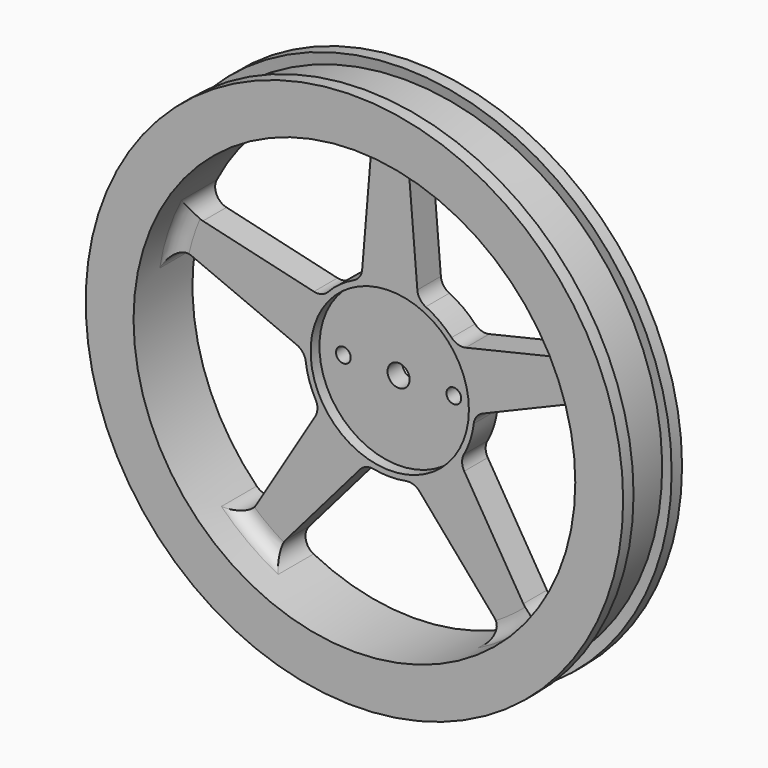
from build123d import *

# Parameters (mm, degrees)
F0_R          = 36.5
F0_R_2        = 30
F1_DEPTH      = 10
F2_R          = 11.5
F2_R_2        = 1
F2_R_3        = 1.5
F3_DEPTH      = 4
F5_DEPTH      = 4
F6_T1_DEPTH   = 4
F6_T6_ANGLE   = 27.7282501568
F6_T12_ANGLE  = 27.7282501568
F6_T18_ANGLE  = 27.7282501568
F6_T24_ANGLE  = 27.7282501568
F6_T30_ANGLE  = 27.7282501568
F6_T37_ANGLE  = 27.7282501568
F6_T41_DEPTH  = 10.3294220662
F6_T49_DEPTH  = 10.3294220662
F6_T54_ANGLE  = 27.7282501568
F6_T61_ANGLE  = 27.7282501568
F6_T65_DEPTH  = 10.3294220662
F6_T73_DEPTH  = 10.3294220662
F6_T78_ANGLE  = 27.7282501568
F6_T85_ANGLE  = 27.7282501568
F6_T89_DEPTH  = 10.3294220662
F6_T97_DEPTH  = 10.3294220662
F6_T102_ANGLE = 27.7282501568
F6_T109_ANGLE = 27.7282501568
F6_T113_DEPTH = 10.3294220662
F6_T121_DEPTH = 10.3294220662
F6_T126_ANGLE = 27.7282501568
F6_T133_ANGLE = 27.7282501568
F6_T137_DEPTH = 10.3294220662
F6_T145_DEPTH = 10.3294220662
F6_T150_ANGLE = 27.7282501568
F7_R          = 10.75
F8_DEPTH      = 1.5


# Not quite as in the source:
# - a fillet or chamfer that OpenCascade refuses, or shapes differently, is made with other operations: its cross-section is extruded or revolved along the edge and cut away or added
# - a feature names something its author has since deleted; it is built from what else it names


with BuildPart() as f1:
    # F0 (on Front) → F1 (new body)
    with BuildSketch(Plane.XZ):
        Circle(F0_R)
        Circle(F0_R_2, mode=Mode.SUBTRACT)
    extrude(amount=F1_DEPTH)



with BuildPart() as f3:
    # F2 (on Front) → F3 (new body)
    with BuildSketch(Plane.XZ):
        Circle(F2_R)
        with Locations((-7.5, 0)):
            Circle(F2_R_2, mode=Mode.SUBTRACT)
        Circle(F2_R_3, mode=Mode.SUBTRACT)
        with Locations((7.5, 0)):
            Circle(F2_R_2, mode=Mode.SUBTRACT)
    extrude(amount=F3_DEPTH)


with BuildPart() as f1_1:
    add(f1.part)

    add(f3.part)  # F5 merges F3
    # F4 (on Front) → F5 (join)
    with BuildSketch(Plane.XZ):
        Polygon((-2, 33), (-4, 9), (4, 9), (2, 33), align=None)
        Polygon((-30.766831049, 12.099673847), (-32.0028990265, 8.2954477818), (-9.7955766242, -1.0230731158), (-7.3234406692, 6.5853790146), align=None)
        Polygon((-21.0149473144, -25.5219903098), (-17.7788793369, -27.873131319), (-2.0539992931, -9.6322939585), (-8.5261352481, -4.9300119402), align=None)
        Polygon((17.7788793369, -27.873131319), (21.0149473144, -25.5219903098), (8.5261352481, -4.9300119402), (2.0539992931, -9.6322939585), align=None)
        Polygon((32.0028990265, 8.2954477818), (30.766831049, 12.099673847), (7.3234406692, 6.5853790146), (9.7955766242, -1.0230731158), align=None)
    extrude(amount=F5_DEPTH)

    # F6: fillet of radius 2 on 25 edges, made by hand

    # F6_s2 → F6_t1 (join)
    with BuildSketch(Plane.XZ):
        with BuildLine():
            ThreePointArc((4.7713926974, 29.6181331574), (3.0942624237, 29.1109072971), (2.4602083344, 27.4774999872))
            Line((2.4602083344, 27.4774999872), (2.2570856463, 29.9149722444))
            ThreePointArc((2.2570856463, 29.9149722444), (3.5173719334, 29.7930880354), (4.7713926974, 29.6181331574))
        make_face()
        with BuildLine():
            ThreePointArc((-4.7713926974, 29.6181331574), (-3.0942624237, 29.1109072971), (-2.4602083344, 27.4774999872))
            Line((-2.4602083344, 27.4774999872), (-2.2570856463, 29.9149722444))
            ThreePointArc((-2.2570856463, 29.9149722444), (-3.5173719334, 29.7930880354), (-4.7713926974, 29.6181331574))
        make_face()
        with BuildLine():
            ThreePointArc((-13.5489640913, -26.7661273264), (-14.6076511042, -25.3699805444), (-14.1605189101, -23.6758386291))
            Line((-14.1605189101, -23.6758386291), (-15.7575588624, -25.5284025881))
            ThreePointArc((-15.7575588624, -25.5284025881), (-14.6663240978, -26.1705738848), (-13.5489640913, -26.7661273264))
        make_face()
        with BuildLine():
            ThreePointArc((-26.6940771095, 13.6903706039), (-26.7299384062, 11.9385835177), (-25.3724092293, 10.8308116268))
            Line((-25.3724092293, 10.8308116268), (-27.7533514654, 11.3908508215))
            ThreePointArc((-27.7533514654, 11.3908508215), (-27.2479828136, 12.5517900153), (-26.6940771095, 13.6903706039))
        make_face()
        with BuildLine():
            ThreePointArc((-29.6429599701, 4.6146423706), (-28.6422977541, 6.0529466353), (-26.8929015993, 6.1512172911))
            Line((-26.8929015993, 6.1512172911), (-29.1483071103, 7.097618798))
            ThreePointArc((-29.1483071103, 7.097618798), (-29.4218382195, 5.8613510203), (-29.6429599701, 4.6146423706))
        make_face()
        with BuildLine():
            ThreePointArc((-21.2692396494, -21.1570188055), (-19.6142728759, -21.7324569056), (-18.1412196146, -20.783690276))
            Line((-18.1412196146, -20.783690276), (-19.4096001536, -22.8750392759))
            ThreePointArc((-19.4096001536, -22.8750392759), (-20.3575514371, -22.0356551862), (-21.2692396494, -21.1570188055))
        make_face()
        with BuildLine():
            ThreePointArc((-4.054653915, -11.9530503313), (-3.1974418623, -11.3701338379), (-2.1635629978, -11.2946445342))
            ThreePointArc((-2.1635629978, -11.2946445342), (-2.7140069187, -11.1751584528), (-3.2579399845, -11.028863362))
            Line((-3.2579399845, -11.028863362), (-4.054653915, -11.9530503313))
        make_face()
        with BuildLine():
            ThreePointArc((-10.1150694411, -7.5499007142), (-9.8255760037, -6.5545125029), (-10.0732675488, -5.547907794))
            ThreePointArc((-10.0732675488, -5.547907794), (-9.7895330065, -6.034487842), (-9.4823135459, -6.5065912594))
            Line((-9.4823135459, -6.5065912594), (-10.1150694411, -7.5499007142))
        make_face()
        with BuildLine():
            ThreePointArc((-12.6209833732, 0.1625093402), (-11.8017037517, -0.4726166656), (-11.4104230182, -1.432566419))
            ThreePointArc((-11.4104230182, -1.432566419), (-11.4668815279, -0.8721399115), (-11.4958311896, -0.3096211556))
            Line((-11.4958311896, -0.3096211556), (-12.6209833732, 0.1625093402))
        make_face()
        with BuildLine():
            ThreePointArc((-10.3061106282, 7.2869550782), (-9.2699817917, 7.3192223314), (-8.3891847207, 7.8658489511))
            ThreePointArc((-8.3891847207, 7.8658489511), (-8.7642710506, 7.4456398617), (-9.1183320478, 7.0075688128))
            Line((-9.1183320478, 7.0075688128), (-10.3061106282, 7.2869550782))
        make_face()
        with BuildLine():
            ThreePointArc((-3.7455427811, 12.053486627), (-4.0964121814, 11.0780406749), (-4.8884662535, 10.4092697961))
            ThreePointArc((-4.8884662535, 10.4092697961), (-4.3729156105, 10.6361463446), (-3.8468744196, 10.8375069642))
            Line((-3.8468744196, 10.8375069642), (-3.7455427811, 12.053486627))
        make_face()
        with BuildLine():
            ThreePointArc((3.7455427811, 12.053486627), (4.0964121814, 11.0780406749), (4.8884662535, 10.4092697961))
            ThreePointArc((4.8884662535, 10.4092697961), (4.3729156105, 10.6361463446), (3.8468744196, 10.8375069642))
            Line((3.8468744196, 10.8375069642), (3.7455427811, 12.053486627))
        make_face()
        with BuildLine():
            ThreePointArc((29.6429599701, 4.6146423706), (28.6422977541, 6.0529466353), (26.8929015993, 6.1512172911))
            Line((26.8929015993, 6.1512172911), (29.1483071103, 7.097618798))
            ThreePointArc((29.1483071103, 7.097618798), (29.4218382195, 5.8613510203), (29.6429599701, 4.6146423706))
        make_face()
        with BuildLine():
            ThreePointArc((26.6940771095, 13.6903706039), (26.7299384062, 11.9385835177), (25.3724092293, 10.8308116268))
            Line((25.3724092293, 10.8308116268), (27.7533514654, 11.3908508215))
            ThreePointArc((27.7533514654, 11.3908508215), (27.2479828136, 12.5517900153), (26.6940771095, 13.6903706039))
        make_face()
        with BuildLine():
            ThreePointArc((13.5489640913, -26.7661273264), (14.6076511042, -25.3699805444), (14.1605189101, -23.6758386291))
            Line((14.1605189101, -23.6758386291), (15.7575588624, -25.5284025881))
            ThreePointArc((15.7575588624, -25.5284025881), (14.6663240978, -26.1705738848), (13.5489640913, -26.7661273264))
        make_face()
        with BuildLine():
            ThreePointArc((21.2692396494, -21.1570188055), (19.6142728759, -21.7324569056), (18.1412196146, -20.783690276))
            Line((18.1412196146, -20.783690276), (19.4096001536, -22.8750392759))
            ThreePointArc((19.4096001536, -22.8750392759), (20.3575514371, -22.0356551862), (21.2692396494, -21.1570188055))
        make_face()
        with BuildLine():
            ThreePointArc((12.6209833732, 0.1625093402), (11.8017037517, -0.4726166656), (11.4104230182, -1.432566419))
            ThreePointArc((11.4104230182, -1.432566419), (11.4668815279, -0.8721399115), (11.4958311896, -0.3096211556))
            Line((11.4958311896, -0.3096211556), (12.6209833732, 0.1625093402))
        make_face()
        with BuildLine():
            ThreePointArc((10.3061106282, 7.2869550782), (9.2699817917, 7.3192223314), (8.3891847207, 7.8658489511))
            ThreePointArc((8.3891847207, 7.8658489511), (8.7642710506, 7.4456398617), (9.1183320478, 7.0075688128))
            Line((9.1183320478, 7.0075688128), (10.3061106282, 7.2869550782))
        make_face()
        with BuildLine():
            ThreePointArc((4.054653915, -11.9530503313), (3.1974418623, -11.3701338379), (2.1635629978, -11.2946445342))
            ThreePointArc((2.1635629978, -11.2946445342), (2.7140069187, -11.1751584528), (3.2579399845, -11.028863362))
            Line((3.2579399845, -11.028863362), (4.054653915, -11.9530503313))
        make_face()
        with BuildLine():
            ThreePointArc((10.1150694411, -7.5499007142), (9.8255760037, -6.5545125029), (10.0732675488, -5.547907794))
            ThreePointArc((10.0732675488, -5.547907794), (9.7895330065, -6.034487842), (9.4823135459, -6.5065912594))
            Line((9.4823135459, -6.5065912594), (10.1150694411, -7.5499007142))
        make_face()
    extrude(amount=F6_T1_DEPTH)


with BuildPart() as f6_tool4:
    # F6_s5 → F6_t6 (revolve)
    with BuildSketch(Plane(origin=(0, 0, 0), x_dir=(0, 1, 0), z_dir=(-0.5279066599, 0, 0.8493023952))):
        with BuildLine():
            ThreePointArc((-6, -30), (-4.5857864376, -29.4142135624), (-4, -28))
            Line((-4, -28), (-4, -30))
            Line((-4, -30), (-6, -30))
        make_face()
    revolve(axis=Axis((0, -4, 0), (0, 1, 0)), revolution_arc=F6_T6_ANGLE)

    split(bisect_by=Plane(origin=(1.8315713488, 0, -4.3648875067), x_dir=(0, 1, 0), z_dir=(-0.3869305197, 0, 0.9221088726)), keep=Keep.TOP)

    split(bisect_by=Plane(origin=(-1.0838441567, 0, 4.6078387988), x_dir=(0, 1, 0), z_dir=(0.2289686302, 0, -0.9734338017)), keep=Keep.TOP)


with BuildPart() as f1_2:
    add(f1_1.part)

    # F6_t3: union F6_tool4
    add(f6_tool4.part)


with BuildPart() as f6_tool10:
    # F6_s11 → F6_t12 (revolve)
    with BuildSketch(Plane(origin=(0, 0, 0), x_dir=(0, 1, 0), z_dir=(-0.9708667066, 0, -0.2396201954))):
        with BuildLine():
            ThreePointArc((-6, -30), (-4.5857864376, -29.4142135624), (-4, -28))
            Line((-4, -28), (-4, -30))
            Line((-4, -30), (-6, -30))
        make_face()
    revolve(axis=Axis((0, -4, 0), (0, 1, 0)), revolution_arc=F6_T12_ANGLE)

    split(bisect_by=Plane(origin=(4.7172413793, 0, 0.3931034483), x_dir=(0, 1, 0), z_dir=(-0.9965457582, 0, -0.0830454799)), keep=Keep.TOP)

    split(bisect_by=Plane(origin=(-4.7172413793, 0, 0.3931034483), x_dir=(0, 1, 0), z_dir=(0.9965457582, 0, -0.0830454799)), keep=Keep.TOP)


with BuildPart() as f1_3:
    add(f1_2.part)

    # F6_t9: union F6_tool10
    add(f6_tool10.part)


with BuildPart() as f6_tool16:
    # F6_s17 → F6_t18 (revolve)
    with BuildSketch(Plane(origin=(0, 0, 0), x_dir=(0, 1, 0), z_dir=(-0.0721219634, 0, -0.9973958203))):
        with BuildLine():
            ThreePointArc((-6, -30), (-4.5857864376, -29.4142135624), (-4, -28))
            Line((-4, -28), (-4, -30))
            Line((-4, -30), (-6, -30))
        make_face()
    revolve(axis=Axis((0, -4, 0), (0, 1, 0)), revolution_arc=F6_T18_ANGLE)

    split(bisect_by=Plane(origin=(1.0838441567, 0, 4.6078387988), x_dir=(0, 1, 0), z_dir=(-0.2289686302, 0, -0.9734338017)), keep=Keep.TOP)

    split(bisect_by=Plane(origin=(-1.8315713488, 0, -4.3648875067), x_dir=(0, 1, 0), z_dir=(0.3869305197, 0, 0.9221088726)), keep=Keep.TOP)


with BuildPart() as f1_4:
    add(f1_3.part)

    # F6_t15: union F6_tool16
    add(f6_tool16.part)


with BuildPart() as f6_tool22:
    # F6_s23 → F6_t24 (revolve)
    with BuildSketch(Plane(origin=(0, 0, 0), x_dir=(0, 1, 0), z_dir=(0.9262928819, 0, -0.3768043218))):
        with BuildLine():
            ThreePointArc((-6, -30), (-4.5857864376, -29.4142135624), (-4, -28))
            Line((-4, -28), (-4, -30))
            Line((-4, -30), (-6, -30))
        make_face()
    revolve(axis=Axis((0, -4, 0), (0, 1, 0)), revolution_arc=F6_T24_ANGLE)

    split(bisect_by=Plane(origin=(-4.047388852, 0, 2.4546975441), x_dir=(0, 1, 0), z_dir=(0.8550353624, 0, -0.5185696954)), keep=Keep.TOP)

    split(bisect_by=Plane(origin=(3.5852680329, 0, -3.0907522845), x_dir=(0, 1, 0), z_dir=(-0.7574095458, 0, 0.6529401044)), keep=Keep.TOP)


with BuildPart() as f1_5:
    add(f1_4.part)

    # F6_t21: union F6_tool22
    add(f6_tool22.part)


with BuildPart() as f6_tool28:
    # F6_s29 → F6_t30 (revolve)
    with BuildSketch(Plane(origin=(0, 0, 0), x_dir=(0, 1, 0), z_dir=(0.6446024479, 0, 0.7645179423))):
        with BuildLine():
            ThreePointArc((-6, -30), (-4.5857864376, -29.4142135624), (-4, -28))
            Line((-4, -28), (-4, -30))
            Line((-4, -30), (-6, -30))
        make_face()
    revolve(axis=Axis((0, -4, 0), (0, 1, 0)), revolution_arc=F6_T30_ANGLE)

    split(bisect_by=Plane(origin=(-3.5852680329, 0, -3.0907522845), x_dir=(0, 1, 0), z_dir=(0.7574095458, 0, 0.6529401044)), keep=Keep.TOP)

    split(bisect_by=Plane(origin=(4.047388852, 0, 2.4546975441), x_dir=(0, 1, 0), z_dir=(-0.8550353624, 0, -0.5185696954)), keep=Keep.TOP)


with BuildPart() as f1_6:
    add(f1_5.part)

    # F6_t27: union F6_tool28
    add(f6_tool28.part)


with BuildPart() as f6_tool35:
    # F6_s36 → F6_t37 (revolve)
    with BuildSketch(Plane(origin=(0, 0, 0), x_dir=(0, 1, 0), z_dir=(-0.5279066599, 0, 0.8493023952))):
        with BuildLine():
            ThreePointArc((-6, -30), (-4.5857864376, -29.4142135624), (-4, -28))
            Line((-4, -28), (-4, -30))
            Line((-4, -30), (-6, -30))
        make_face()
    revolve(axis=Axis((0, -4, 0), (0, 1, 0)), revolution_arc=F6_T37_ANGLE)

    split(bisect_by=Plane(origin=(-1.0838441567, 0, 4.6078387988), x_dir=(0, 1, 0), z_dir=(-0.2289686302, 0, 0.9734338017)), keep=Keep.TOP)


with BuildPart() as f6_tool39:
    # F6_s40 → F6_t41 (new body)
    with BuildSketch(Plane.XZ.offset(10.3294220662)):
        with BuildLine():
            ThreePointArc((26.6940771095, 13.6903706039), (26.7299384062, 11.9385835177), (25.3724092293, 10.8308116268))
            Line((25.3724092293, 10.8308116268), (27.7533514654, 11.3908508215))
            ThreePointArc((27.7533514654, 11.3908508215), (27.2479828136, 12.5517900153), (26.6940771095, 13.6903706039))
        make_face()
    extrude(amount=-F6_T41_DEPTH)

    split(bisect_by=Plane.XZ.offset(10), keep=Keep.BOTTOM)

    split(bisect_by=Plane.XZ.offset(4), keep=Keep.TOP)


with BuildPart() as f6_tool35_1:
    add(f6_tool35.part)

    # F6_t44: intersect F6_tool39
    add(f6_tool39.part, mode=Mode.INTERSECT)


with BuildPart() as f1_7:
    add(f1_6.part)

    # F6_t33: union F6_tool35
    add(f6_tool35_1.part)


with BuildPart() as f6_tool47:
    # F6_s48 → F6_t49 (new body)
    with BuildSketch(Plane.XZ.offset(10.3294220662)):
        with BuildLine():
            ThreePointArc((29.6429599701, 4.6146423706), (28.6422977541, 6.0529466353), (26.8929015993, 6.1512172911))
            Line((26.8929015993, 6.1512172911), (29.1483071103, 7.097618798))
            ThreePointArc((29.1483071103, 7.097618798), (29.4218382195, 5.8613510203), (29.6429599701, 4.6146423706))
        make_face()
    extrude(amount=-F6_T49_DEPTH)

    split(bisect_by=Plane.XZ.offset(10), keep=Keep.BOTTOM)

    split(bisect_by=Plane.XZ.offset(4), keep=Keep.TOP)


with BuildPart() as f6_tool52:
    # F6_s53 → F6_t54 (revolve)
    with BuildSketch(Plane(origin=(0, 0, 0), x_dir=(0, 1, 0), z_dir=(-0.5279066599, 0, 0.8493023952))):
        with BuildLine():
            ThreePointArc((-6, -30), (-4.5857864376, -29.4142135624), (-4, -28))
            Line((-4, -28), (-4, -30))
            Line((-4, -30), (-6, -30))
        make_face()
    revolve(axis=Axis((0, -4, 0), (0, 1, 0)), revolution_arc=F6_T54_ANGLE)

    split(bisect_by=Plane(origin=(1.8315713488, 0, -4.3648875067), x_dir=(0, 1, 0), z_dir=(0.3869305197, 0, -0.9221088726)), keep=Keep.TOP)


with BuildPart() as f6_tool47_1:
    add(f6_tool47.part)

    # F6_t56: intersect F6_tool52
    add(f6_tool52.part, mode=Mode.INTERSECT)


with BuildPart() as f1_8:
    add(f1_7.part)

    # F6_t45: union F6_tool47
    add(f6_tool47_1.part)


with BuildPart() as f6_tool59:
    # F6_s60 → F6_t61 (revolve)
    with BuildSketch(Plane(origin=(0, 0, 0), x_dir=(0, 1, 0), z_dir=(-0.9708667066, 0, -0.2396201954))):
        with BuildLine():
            ThreePointArc((-6, -30), (-4.5857864376, -29.4142135624), (-4, -28))
            Line((-4, -28), (-4, -30))
            Line((-4, -30), (-6, -30))
        make_face()
    revolve(axis=Axis((0, -4, 0), (0, 1, 0)), revolution_arc=F6_T61_ANGLE)

    split(bisect_by=Plane(origin=(-4.7172413793, 0, 0.3931034483), x_dir=(0, 1, 0), z_dir=(-0.9965457582, 0, 0.0830454799)), keep=Keep.TOP)


with BuildPart() as f6_tool63:
    # F6_s64 → F6_t65 (new body)
    with BuildSketch(Plane.XZ.offset(10.3294220662)):
        with BuildLine():
            ThreePointArc((-4.7713926974, 29.6181331574), (-3.0942624237, 29.1109072971), (-2.4602083344, 27.4774999872))
            Line((-2.4602083344, 27.4774999872), (-2.2570856463, 29.9149722444))
            ThreePointArc((-2.2570856463, 29.9149722444), (-3.5173719334, 29.7930880354), (-4.7713926974, 29.6181331574))
        make_face()
    extrude(amount=-F6_T65_DEPTH)

    split(bisect_by=Plane.XZ.offset(10), keep=Keep.BOTTOM)

    split(bisect_by=Plane.XZ.offset(4), keep=Keep.TOP)


with BuildPart() as f6_tool59_1:
    add(f6_tool59.part)

    # F6_t68: intersect F6_tool63
    add(f6_tool63.part, mode=Mode.INTERSECT)


with BuildPart() as f1_9:
    add(f1_8.part)

    # F6_t57: union F6_tool59
    add(f6_tool59_1.part)


with BuildPart() as f6_tool71:
    # F6_s72 → F6_t73 (new body)
    with BuildSketch(Plane.XZ.offset(10.3294220662)):
        with BuildLine():
            ThreePointArc((4.7713926974, 29.6181331574), (3.0942624237, 29.1109072971), (2.4602083344, 27.4774999872))
            Line((2.4602083344, 27.4774999872), (2.2570856463, 29.9149722444))
            ThreePointArc((2.2570856463, 29.9149722444), (3.5173719334, 29.7930880354), (4.7713926974, 29.6181331574))
        make_face()
    extrude(amount=-F6_T73_DEPTH)

    split(bisect_by=Plane.XZ.offset(10), keep=Keep.BOTTOM)

    split(bisect_by=Plane.XZ.offset(4), keep=Keep.TOP)


with BuildPart() as f6_tool76:
    # F6_s77 → F6_t78 (revolve)
    with BuildSketch(Plane(origin=(0, 0, 0), x_dir=(0, 1, 0), z_dir=(-0.9708667066, 0, -0.2396201954))):
        with BuildLine():
            ThreePointArc((-6, -30), (-4.5857864376, -29.4142135624), (-4, -28))
            Line((-4, -28), (-4, -30))
            Line((-4, -30), (-6, -30))
        make_face()
    revolve(axis=Axis((0, -4, 0), (0, 1, 0)), revolution_arc=F6_T78_ANGLE)

    split(bisect_by=Plane(origin=(4.7172413793, 0, 0.3931034483), x_dir=(0, 1, 0), z_dir=(0.9965457582, 0, 0.0830454799)), keep=Keep.TOP)


with BuildPart() as f6_tool71_1:
    add(f6_tool71.part)

    # F6_t80: intersect F6_tool76
    add(f6_tool76.part, mode=Mode.INTERSECT)


with BuildPart() as f1_10:
    add(f1_9.part)

    # F6_t69: union F6_tool71
    add(f6_tool71_1.part)


with BuildPart() as f6_tool83:
    # F6_s84 → F6_t85 (revolve)
    with BuildSketch(Plane(origin=(0, 0, 0), x_dir=(0, 1, 0), z_dir=(-0.0721219634, 0, -0.9973958203))):
        with BuildLine():
            ThreePointArc((-6, -30), (-4.5857864376, -29.4142135624), (-4, -28))
            Line((-4, -28), (-4, -30))
            Line((-4, -30), (-6, -30))
        make_face()
    revolve(axis=Axis((0, -4, 0), (0, 1, 0)), revolution_arc=F6_T85_ANGLE)

    split(bisect_by=Plane(origin=(-1.8315713488, 0, -4.3648875067), x_dir=(0, 1, 0), z_dir=(-0.3869305197, 0, -0.9221088726)), keep=Keep.TOP)


with BuildPart() as f6_tool87:
    # F6_s88 → F6_t89 (new body)
    with BuildSketch(Plane.XZ.offset(10.3294220662)):
        with BuildLine():
            ThreePointArc((-29.6429599701, 4.6146423706), (-28.6422977541, 6.0529466353), (-26.8929015993, 6.1512172911))
            Line((-26.8929015993, 6.1512172911), (-29.1483071103, 7.097618798))
            ThreePointArc((-29.1483071103, 7.097618798), (-29.4218382195, 5.8613510203), (-29.6429599701, 4.6146423706))
        make_face()
    extrude(amount=-F6_T89_DEPTH)

    split(bisect_by=Plane.XZ.offset(10), keep=Keep.BOTTOM)

    split(bisect_by=Plane.XZ.offset(4), keep=Keep.TOP)


with BuildPart() as f6_tool83_1:
    add(f6_tool83.part)

    # F6_t92: intersect F6_tool87
    add(f6_tool87.part, mode=Mode.INTERSECT)


with BuildPart() as f1_11:
    add(f1_10.part)

    # F6_t81: union F6_tool83
    add(f6_tool83_1.part)


with BuildPart() as f6_tool95:
    # F6_s96 → F6_t97 (new body)
    with BuildSketch(Plane.XZ.offset(10.3294220662)):
        with BuildLine():
            ThreePointArc((-26.6940771095, 13.6903706039), (-26.7299384062, 11.9385835177), (-25.3724092293, 10.8308116268))
            Line((-25.3724092293, 10.8308116268), (-27.7533514654, 11.3908508215))
            ThreePointArc((-27.7533514654, 11.3908508215), (-27.2479828136, 12.5517900153), (-26.6940771095, 13.6903706039))
        make_face()
    extrude(amount=-F6_T97_DEPTH)

    split(bisect_by=Plane.XZ.offset(10), keep=Keep.BOTTOM)

    split(bisect_by=Plane.XZ.offset(4), keep=Keep.TOP)


with BuildPart() as f6_tool100:
    # F6_s101 → F6_t102 (revolve)
    with BuildSketch(Plane(origin=(0, 0, 0), x_dir=(0, 1, 0), z_dir=(-0.0721219634, 0, -0.9973958203))):
        with BuildLine():
            ThreePointArc((-6, -30), (-4.5857864376, -29.4142135624), (-4, -28))
            Line((-4, -28), (-4, -30))
            Line((-4, -30), (-6, -30))
        make_face()
    revolve(axis=Axis((0, -4, 0), (0, 1, 0)), revolution_arc=F6_T102_ANGLE)

    split(bisect_by=Plane(origin=(1.0838441567, 0, 4.6078387988), x_dir=(0, 1, 0), z_dir=(0.2289686302, 0, 0.9734338017)), keep=Keep.TOP)


with BuildPart() as f6_tool95_1:
    add(f6_tool95.part)

    # F6_t104: intersect F6_tool100
    add(f6_tool100.part, mode=Mode.INTERSECT)


with BuildPart() as f1_12:
    add(f1_11.part)

    # F6_t93: union F6_tool95
    add(f6_tool95_1.part)


with BuildPart() as f6_tool107:
    # F6_s108 → F6_t109 (revolve)
    with BuildSketch(Plane(origin=(0, 0, 0), x_dir=(0, 1, 0), z_dir=(0.9262928819, 0, -0.3768043218))):
        with BuildLine():
            ThreePointArc((-6, -30), (-4.5857864376, -29.4142135624), (-4, -28))
            Line((-4, -28), (-4, -30))
            Line((-4, -30), (-6, -30))
        make_face()
    revolve(axis=Axis((0, -4, 0), (0, 1, 0)), revolution_arc=F6_T109_ANGLE)

    split(bisect_by=Plane(origin=(3.5852680329, 0, -3.0907522845), x_dir=(0, 1, 0), z_dir=(0.7574095458, 0, -0.6529401044)), keep=Keep.TOP)


with BuildPart() as f6_tool111:
    # F6_s112 → F6_t113 (new body)
    with BuildSketch(Plane.XZ.offset(10.3294220662)):
        with BuildLine():
            ThreePointArc((-13.5489640913, -26.7661273264), (-14.6076511042, -25.3699805444), (-14.1605189101, -23.6758386291))
            Line((-14.1605189101, -23.6758386291), (-15.7575588624, -25.5284025881))
            ThreePointArc((-15.7575588624, -25.5284025881), (-14.6663240978, -26.1705738848), (-13.5489640913, -26.7661273264))
        make_face()
    extrude(amount=-F6_T113_DEPTH)

    split(bisect_by=Plane.XZ.offset(10), keep=Keep.BOTTOM)

    split(bisect_by=Plane.XZ.offset(4), keep=Keep.TOP)


with BuildPart() as f6_tool107_1:
    add(f6_tool107.part)

    # F6_t116: intersect F6_tool111
    add(f6_tool111.part, mode=Mode.INTERSECT)


with BuildPart() as f1_13:
    add(f1_12.part)

    # F6_t105: union F6_tool107
    add(f6_tool107_1.part)


with BuildPart() as f6_tool119:
    # F6_s120 → F6_t121 (new body)
    with BuildSketch(Plane.XZ.offset(10.3294220662)):
        with BuildLine():
            ThreePointArc((-21.2692396494, -21.1570188055), (-19.6142728759, -21.7324569056), (-18.1412196146, -20.783690276))
            Line((-18.1412196146, -20.783690276), (-19.4096001536, -22.8750392759))
            ThreePointArc((-19.4096001536, -22.8750392759), (-20.3575514371, -22.0356551862), (-21.2692396494, -21.1570188055))
        make_face()
    extrude(amount=-F6_T121_DEPTH)

    split(bisect_by=Plane.XZ.offset(10), keep=Keep.BOTTOM)

    split(bisect_by=Plane.XZ.offset(4), keep=Keep.TOP)


with BuildPart() as f6_tool124:
    # F6_s125 → F6_t126 (revolve)
    with BuildSketch(Plane(origin=(0, 0, 0), x_dir=(0, 1, 0), z_dir=(0.9262928819, 0, -0.3768043218))):
        with BuildLine():
            ThreePointArc((-6, -30), (-4.5857864376, -29.4142135624), (-4, -28))
            Line((-4, -28), (-4, -30))
            Line((-4, -30), (-6, -30))
        make_face()
    revolve(axis=Axis((0, -4, 0), (0, 1, 0)), revolution_arc=F6_T126_ANGLE)

    split(bisect_by=Plane(origin=(-4.047388852, 0, 2.4546975441), x_dir=(0, 1, 0), z_dir=(-0.8550353624, 0, 0.5185696954)), keep=Keep.TOP)


with BuildPart() as f6_tool119_1:
    add(f6_tool119.part)

    # F6_t128: intersect F6_tool124
    add(f6_tool124.part, mode=Mode.INTERSECT)


with BuildPart() as f1_14:
    add(f1_13.part)

    # F6_t117: union F6_tool119
    add(f6_tool119_1.part)


with BuildPart() as f6_tool131:
    # F6_s132 → F6_t133 (revolve)
    with BuildSketch(Plane(origin=(0, 0, 0), x_dir=(0, 1, 0), z_dir=(0.6446024479, 0, 0.7645179423))):
        with BuildLine():
            ThreePointArc((-6, -30), (-4.5857864376, -29.4142135624), (-4, -28))
            Line((-4, -28), (-4, -30))
            Line((-4, -30), (-6, -30))
        make_face()
    revolve(axis=Axis((0, -4, 0), (0, 1, 0)), revolution_arc=F6_T133_ANGLE)

    split(bisect_by=Plane(origin=(4.047388852, 0, 2.4546975441), x_dir=(0, 1, 0), z_dir=(0.8550353624, 0, 0.5185696954)), keep=Keep.TOP)


with BuildPart() as f6_tool135:
    # F6_s136 → F6_t137 (new body)
    with BuildSketch(Plane.XZ.offset(10.3294220662)):
        with BuildLine():
            ThreePointArc((21.2692396494, -21.1570188055), (19.6142728759, -21.7324569056), (18.1412196146, -20.783690276))
            Line((18.1412196146, -20.783690276), (19.4096001536, -22.8750392759))
            ThreePointArc((19.4096001536, -22.8750392759), (20.3575514371, -22.0356551862), (21.2692396494, -21.1570188055))
        make_face()
    extrude(amount=-F6_T137_DEPTH)

    split(bisect_by=Plane.XZ.offset(10), keep=Keep.BOTTOM)

    split(bisect_by=Plane.XZ.offset(4), keep=Keep.TOP)


with BuildPart() as f6_tool131_1:
    add(f6_tool131.part)

    # F6_t140: intersect F6_tool135
    add(f6_tool135.part, mode=Mode.INTERSECT)


with BuildPart() as f1_15:
    add(f1_14.part)

    # F6_t129: union F6_tool131
    add(f6_tool131_1.part)


with BuildPart() as f6_tool143:
    # F6_s144 → F6_t145 (new body)
    with BuildSketch(Plane.XZ.offset(10.3294220662)):
        with BuildLine():
            ThreePointArc((13.5489640913, -26.7661273264), (14.6076511042, -25.3699805444), (14.1605189101, -23.6758386291))
            Line((14.1605189101, -23.6758386291), (15.7575588624, -25.5284025881))
            ThreePointArc((15.7575588624, -25.5284025881), (14.6663240978, -26.1705738848), (13.5489640913, -26.7661273264))
        make_face()
    extrude(amount=-F6_T145_DEPTH)

    split(bisect_by=Plane.XZ.offset(10), keep=Keep.BOTTOM)

    split(bisect_by=Plane.XZ.offset(4), keep=Keep.TOP)


with BuildPart() as f6_tool148:
    # F6_s149 → F6_t150 (revolve)
    with BuildSketch(Plane(origin=(0, 0, 0), x_dir=(0, 1, 0), z_dir=(0.6446024479, 0, 0.7645179423))):
        with BuildLine():
            ThreePointArc((-6, -30), (-4.5857864376, -29.4142135624), (-4, -28))
            Line((-4, -28), (-4, -30))
            Line((-4, -30), (-6, -30))
        make_face()
    revolve(axis=Axis((0, -4, 0), (0, 1, 0)), revolution_arc=F6_T150_ANGLE)

    split(bisect_by=Plane(origin=(-3.5852680329, 0, -3.0907522845), x_dir=(0, 1, 0), z_dir=(-0.7574095458, 0, -0.6529401044)), keep=Keep.TOP)


with BuildPart() as f6_tool143_1:
    add(f6_tool143.part)

    # F6_t152: intersect F6_tool148
    add(f6_tool148.part, mode=Mode.INTERSECT)


with BuildPart() as f1_16:
    add(f1_15.part)

    # F6_t141: union F6_tool143
    add(f6_tool143_1.part)

    # F7 (on face) → F8 (cut)
    with BuildSketch(Plane.XZ.offset(4)):
        Circle(F7_R)
    extrude(amount=-F8_DEPTH, mode=Mode.SUBTRACT)

    # F9 (on Right) → F10 (revolve, cut)
    with BuildSketch(Plane.YZ):
        Polygon((-2.3816349035, 40), (-7.6183650965, 40), (-8.5, 35), (-1.5, 35), align=None)
    revolve(axis=Axis((0, -11.0178330215, 0), (0, -1, 0)), mode=Mode.SUBTRACT)


solid = f1_16.part
